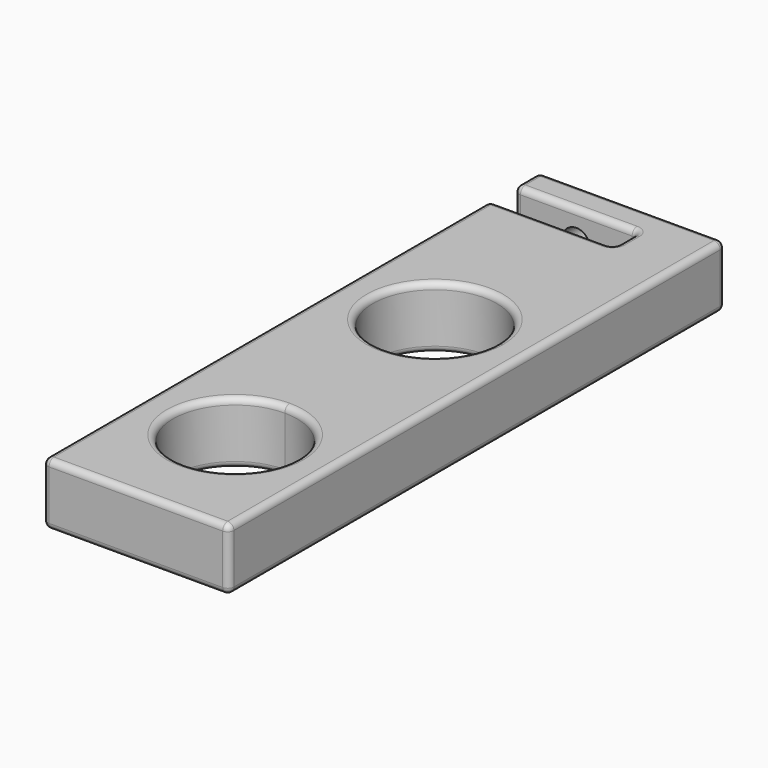
from build123d import *

# Parameters (mm, degrees)
F0_W         = 30
F0_H         = 100
F1_DEPTH     = 10
F2_W         = 20
F2_H         = 5
F3_DEPTH     = 25
F4_R         = 2.25
F5_DEPTH     = 6
F6_R         = 1
F7_F1_R      = 1
F7_F2_R      = 1
F8_T1_DEPTH  = 28
F8_S5_W      = 1
F8_S5_H      = 1
F8_T6_DEPTH  = 1
F8_S11_W     = 1
F8_S11_H     = 1
F8_T12_DEPTH = 1
F10_DEPTH    = 25
F11_R        = 1
F12_R        = 1


# Not quite as in the source:
# - a fillet or chamfer that OpenCascade refuses, or shapes differently, is made with other operations: its cross-section is extruded or revolved along the edge and cut away or added


with BuildPart() as f1:
    # F0 (on Top) → F1 (new body)
    with BuildSketch(Plane.XY):
        Rectangle(F0_W, F0_H)
    extrude(amount=F1_DEPTH)

    # F2 (on face) → F3 (cut)
    with BuildSketch(Plane.XY.offset(10)):
        with Locations((-5, 42.5)):
            Rectangle(F2_W, F2_H)
    extrude(amount=-F3_DEPTH, mode=Mode.SUBTRACT)

    # F4 (on face) → F5 (cut)
    with BuildSketch(Plane(origin=(0, 50, 0), x_dir=(-1, 0, 0), z_dir=(0, 1, 0))):
        with Locations((5, 5)):
            Circle(F4_R)
    extrude(amount=-F5_DEPTH, mode=Mode.SUBTRACT)

    # F6
    f6_edges = [f1.edges().sort_by_distance(p)[0] for p in [
        (-15, 45, 5),
        (-15, 50, 5),
    ]]
    fillet(f6_edges, radius=F6_R)

    # F7: fillet of radius 1 on 19 edges, made by hand

    # F7_f1
    f7_f1_edges = [f1.edges().sort_by_distance(p)[0] for p in [
        (5, 40, 5),
        (5, 45, 5),
    ]]
    fillet(f7_f1_edges, radius=F7_F1_R)

    # F7_f2
    f7_f2_edges = [f1.edges().sort_by_distance(p)[0] for p in [
        (-15, 40, 5),
        (15, 50, 5),
        (15, -50, 5),
        (-15, -50, 5),
        (-15, -5, 10),
        (15, 0, 10),
        (15, 0, 0),
        (0, -50, 0),
        (-5, 45, 0),
        (-14.7071067812, 45.2928932188, 0),
        (5, 42.5, 0),
        (-15, 47.5, 0),
        (-5.5, 40, 0),
        (-14.7071067812, 49.7071067812, 0),
        (-15, -5, 0),
        (0.5, 50, 0),
        (0.5, 50, 10),
        (-14.7071067812, 49.7071067812, 10),
        (-15, 47.5, 10),
        (-14.7071067812, 45.2928932188, 10),
        (-5, 45, 10),
        (4.7071067812, 44.7071067812, 10),
        (4.7071067812, 40.2928932188, 0),
        (4.7071067812, 44.7071067812, 0),
    ]]
    fillet(f7_f2_edges, radius=F7_F2_R)

    # F8: fillet of radius 1 on 1 edges, made by hand

    # F8_s2 → F8_t1 (cut)
    with BuildSketch(Plane.YZ.offset(-14)):
        with BuildLine():
            ThreePointArc((-50, 9), (-49.7071067812, 9.7071067812), (-49, 10))
            Line((-49, 10), (-50, 10))
            Line((-50, 10), (-50, 9))
        make_face()
    extrude(amount=F8_T1_DEPTH, mode=Mode.SUBTRACT)


with BuildPart() as f8_tool4:
    # F8_s5 → F8_t6 (new body)
    with BuildSketch(Plane.XZ.offset(49)):
        with Locations((-14.5, 9.5)):
            Rectangle(F8_S5_W, F8_S5_H)
    extrude(amount=F8_T6_DEPTH)

    # F8_s7 → F8_t8 (revolve, cut)
    with BuildSketch(Plane(origin=(-14, -49, 9), x_dir=(0.7071067812, 0, -0.7071067812), z_dir=(-0.7071067812, 0, -0.7071067812))):
        with BuildLine():
            ThreePointArc((0, -1), (1, 0), (0, 1))
            Line((0, 1), (0, -1))
        make_face()
    revolve(axis=Axis((-14, -49, 9), (0, -1, 0)), mode=Mode.SUBTRACT)


with BuildPart() as f1_1:
    add(f1.part)

    # F8_t3: cut F8_tool4
    add(f8_tool4.part, mode=Mode.SUBTRACT)


with BuildPart() as f8_tool10:
    # F8_s11 → F8_t12 (new body)
    with BuildSketch(Plane.XZ.offset(49)):
        with Locations((14.5, 9.5)):
            Rectangle(F8_S11_W, F8_S11_H)
    extrude(amount=F8_T12_DEPTH)

    # F8_s13 → F8_t14 (revolve, cut)
    with BuildSketch(Plane(origin=(14, -49, 9), x_dir=(-0.7071067812, 0, -0.7071067812), z_dir=(-0.7071067812, 0, 0.7071067812))):
        with BuildLine():
            ThreePointArc((0, -1), (1, 0), (0, 1))
            Line((0, 1), (0, -1))
        make_face()
    revolve(axis=Axis((14, -49, 9), (0, -1, 0)), mode=Mode.SUBTRACT)


with BuildPart() as f1_2:
    add(f1_1.part)

    # F8_t9: cut F8_tool10
    add(f8_tool10.part, mode=Mode.SUBTRACT)

    # F9 (on face) → F10 (cut)
    with BuildSketch(Plane.XY.offset(10)):
        with BuildLine():
            ThreePointArc((0, -20), (-10, -30), (0, -40))
            Line((0, -40), (0, -30))
            Line((0, -30), (0, -20))
        make_face()
        with BuildLine():
            ThreePointArc((10, 10.2520165965), (-7.0710678119, 17.3230844084), (0, 0.2520165965))
            ThreePointArc((0, 0.2520165965), (7.0710678119, 3.1809487846), (10, 10.2520165965))
        make_face()
        with BuildLine():
            Line((0, -30), (0, -40))
            ThreePointArc((0, -40), (7.0710678119, -37.0710678119), (10, -30))
            ThreePointArc((10, -30), (7.0710678119, -22.9289321881), (0, -20))
            Line((0, -20), (0, -30))
        make_face()
    extrude(amount=-F10_DEPTH, mode=Mode.SUBTRACT)

    # F11
    f11_edges = [f1_2.edges().sort_by_distance(p)[0] for p in [
        (0, -20, 0),
    ]]
    fillet(f11_edges, radius=F11_R)

    # F12
    f12_edges = [f1_2.edges().sort_by_distance(p)[0] for p in [
        (0, -20, 10),
        (0, 20.252017, 10),
        (0, 20.252017, 0),
    ]]
    fillet(f12_edges, radius=F12_R)


solid = f1_2.part
